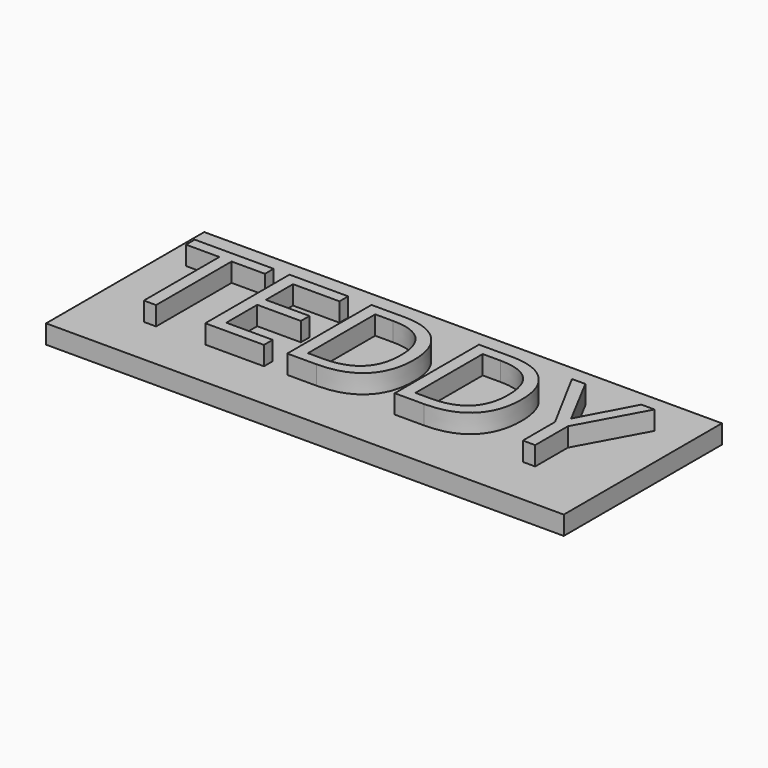
from build123d import *

# Parameters (mm, degrees)
F0_W         = 110
F0_H         = 42
F1_DEPTH     = 4
F2_TEXT_SIZE = 31.3249473839
F3_DEPTH     = 4


# Not quite as in the source:
# - Text() gives the source's letters only with a copy of the font that has no kerning and outlines rounded to 1/6400 em; it was checked with that copy


with BuildPart() as f1:
    # F0 (on Top) → F1 (new body)
    with BuildSketch(Plane.XY):
        Rectangle(F0_W, F0_H)
    extrude(amount=F1_DEPTH)

    # F2 (on face) → F3 (join)
    with BuildSketch(Plane.XY.offset(4)):
        with Locations((-50, -10.4739621164)):
            Text('TEDDY', F2_TEXT_SIZE, font='Open Sans', text_align=(TextAlign.LEFT, TextAlign.BOTTOM))
    extrude(amount=F3_DEPTH)


solid = f1.part
